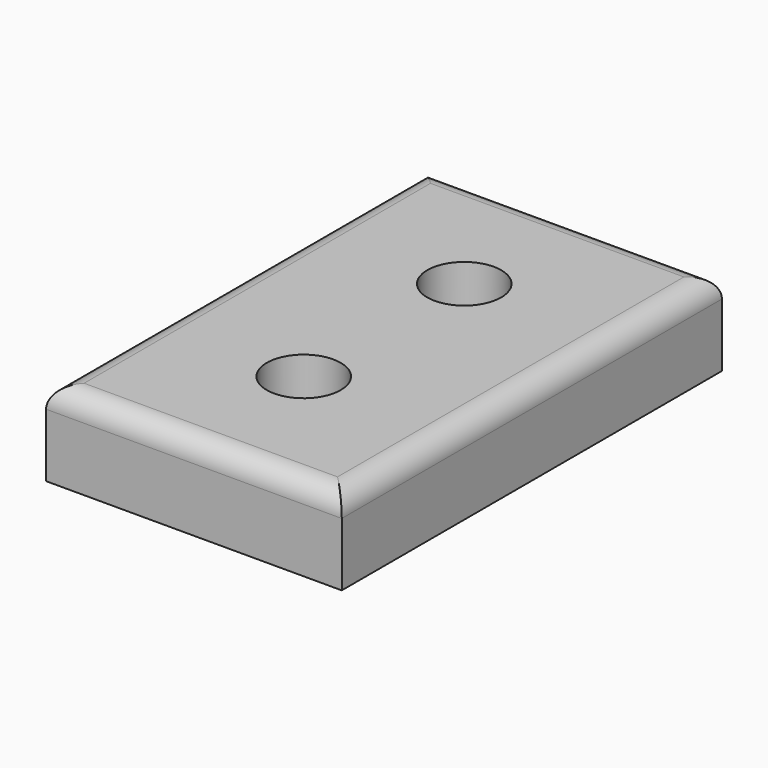
from build123d import *

# Parameters (mm, degrees)
F0_W     = 14
F0_H     = 22.5
F0_R     = 1.75
F1_DEPTH = 4
F2_R     = 1
F3_W     = 1
F3_H     = 6
F4_DEPTH = 0.75
F5_R     = 0.49999


# Not quite as in the source:
# - a fillet or chamfer is up to 0.001 mm smaller than in the source, because OpenCascade refuses the exact size


with BuildPart() as f1:
    # F0 (on Top) → F1 (new body)
    with BuildSketch(Plane.XY):
        with Locations((7, -11.25)):
            Rectangle(F0_W, F0_H)
        with Locations((7, -16)):
            Circle(F0_R, mode=Mode.SUBTRACT)
        with Locations((7, -6.5)):
            Circle(F0_R, mode=Mode.SUBTRACT)
    extrude(amount=F1_DEPTH)

    # F2
    f2_edges = [f1.edges().sort_by_distance(p)[0] for p in [
        (7, 0, 4),
        (0, -11.25, 4),
        (14, -11.25, 4),
        (7, -22.5, 4),
    ]]
    fillet(f2_edges, radius=F2_R)

    # F3 (on face) → F4 (join)
    with BuildSketch(Plane(origin=(0, 0, 0), x_dir=(1, 0, 0), z_dir=(0, 0, -1))):
        with Locations((4, 11.25)):
            Rectangle(F3_W, F3_H)
        with Locations((6, 11.25)):
            Rectangle(F3_W, F3_H)
        with Locations((8, 11.25)):
            Rectangle(F3_W, F3_H)
        with Locations((10, 11.25)):
            Rectangle(F3_W, F3_H)
    extrude(amount=F4_DEPTH)

    # F5 (radius 0.5 in the source; OpenCascade refuses exactly that, so slightly less here)
    f5_edges = [f1.edges().sort_by_distance(p)[0] for p in [
        (10, -8.25, -0.75),
        (10.5, -11.25, -0.75),
        (10, -14.25, -0.75),
        (9.5, -11.25, -0.75),
        (8, -8.25, -0.75),
        (8.5, -11.25, -0.75),
        (8, -14.25, -0.75),
        (7.5, -11.25, -0.75),
        (6, -8.25, -0.75),
        (6.5, -11.25, -0.75),
        (6, -14.25, -0.75),
        (5.5, -11.25, -0.75),
        (4, -8.25, -0.75),
        (4.5, -11.25, -0.75),
        (4, -14.25, -0.75),
        (3.5, -11.25, -0.75),
    ]]
    fillet(f5_edges, radius=F5_R)


solid = f1.part
